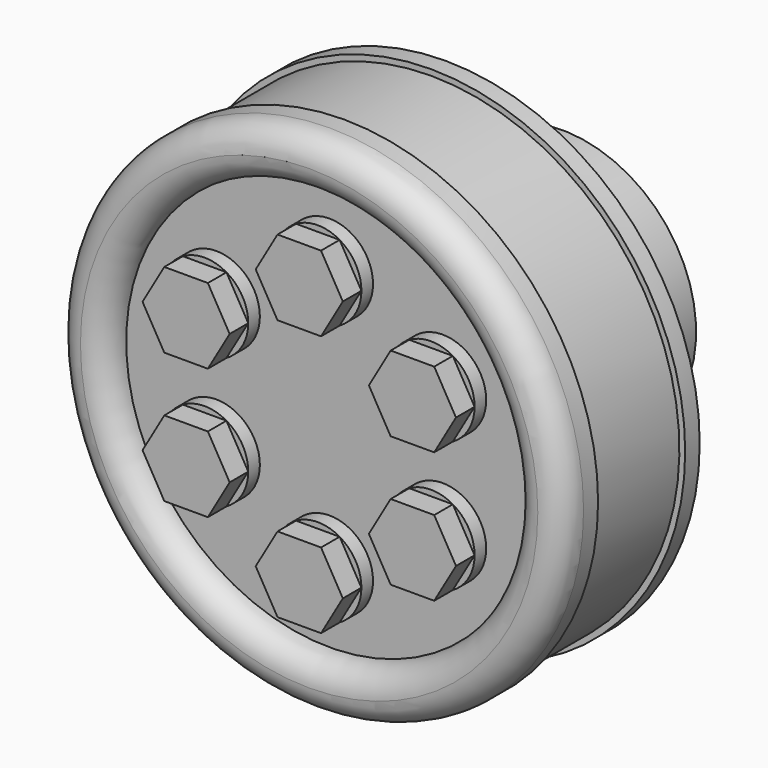
from build123d import *

# Parameters (mm, degrees)
F0_R      = 22.225
F1_DEPTH  = 12.7
F2_R      = 3.81
F3_DEPTH  = 1.27
F5_DEPTH  = 2.032
F6_R      = 22.225
F6_R_2    = 17.78
F7_DEPTH  = 2.2225
F8_R      = 2.22249
F9_R      = 2.2225
F10_R     = 11.7475
F11_DEPTH = 12.7
F12_R     = 3.302
F13_DEPTH = 6.35
F14_R     = 1.7272
F15_DEPTH = 63.5
F16_W     = 9.525
F16_H     = 0.508


# Not quite as in the source:
# - a fillet or chamfer is up to 0.001 mm smaller than in the source, because OpenCascade refuses the exact size


with BuildPart() as f1:
    # F0 (on Front) → F1 (new body)
    with BuildSketch(Plane.XZ):
        Circle(F0_R)
    extrude(amount=F1_DEPTH)

    # F2 (on face) → F3 (join)
    with BuildSketch(Plane.XZ.offset(12.7)):
        with Locations((0, 11.43)):
            Circle(F2_R)
        with Locations((-9.8986703653, 5.715)):
            Circle(F2_R)
        with Locations((-9.8986703653, -5.715)):
            Circle(F2_R)
        with Locations((0, -11.43)):
            Circle(F2_R)
        with Locations((9.8986703653, -5.715)):
            Circle(F2_R)
        with Locations((9.8986703653, 5.715)):
            Circle(F2_R)
    extrude(amount=F3_DEPTH)

    # F4 (on face) → F5 (join)
    with BuildSketch(Plane.XZ.offset(13.97)):
        Polygon((1.905, 8.1304432116), (3.81, 11.43), (1.905, 14.7295567884), (-1.905, 14.7295567884), (-3.81, 11.43), (-1.905, 8.1304432116), align=None)
        Polygon((-7.9936703653, 2.4154432116), (-6.0886703653, 5.715), (-7.9936703653, 9.0145567884), (-11.8036703653, 9.0145567884), (-13.7086703653, 5.715), (-11.8036703653, 2.4154432116), align=None)
        Polygon((7.9936703653, 9.0145567884), (6.0886703653, 5.715), (7.9936703653, 2.4154432116), (11.8036703653, 2.4154432116), (13.7086703653, 5.715), (11.8036703653, 9.0145567884), align=None)
        Polygon((-7.9936703653, -2.4154432116), (-11.8036703653, -2.4154432116), (-13.7086703653, -5.715), (-11.8036703653, -9.0145567884), (-7.9936703653, -9.0145567884), (-6.0886703653, -5.715), align=None)
        Polygon((3.81, -11.43), (1.905, -8.1304432116), (-1.905, -8.1304432116), (-3.81, -11.43), (-1.905, -14.7295567884), (1.905, -14.7295567884), align=None)
        Polygon((7.9936703653, -2.4154432116), (6.0886703653, -5.715), (7.9936703653, -9.0145567884), (11.8036703653, -9.0145567884), (13.7086703653, -5.715), (11.8036703653, -2.4154432116), align=None)
    extrude(amount=F5_DEPTH)

    # F6 (on face) → F7 (join)
    with BuildSketch(Plane.XZ.offset(12.7)):
        Circle(F6_R)
        Circle(F6_R_2, mode=Mode.SUBTRACT)
    extrude(amount=F7_DEPTH)

    # F8 (radius 2.2225 in the source; OpenCascade refuses exactly that, so slightly less here)
    f8_edges = [f1.edges().sort_by_distance(p)[0] for p in [
        (-17.78, -14.9225, 0),
    ]]
    fillet(f8_edges, radius=F8_R)

    # F9
    f9_edges = [f1.edges().sort_by_distance(p)[0] for p in [
        (-22.225, -14.9225, 0),
    ]]
    fillet(f9_edges, radius=F9_R)

    # F10 (on face) → F11 (join)
    with BuildSketch(Plane(origin=(0, 0, 0), x_dir=(-1, 0, 0), z_dir=(0, 1, 0))):
        Circle(F10_R)
    extrude(amount=F11_DEPTH)

    # F12 (on face) → F13 (cut)
    with BuildSketch(Plane(origin=(0, 12.7, 0), x_dir=(-1, 0, 0), z_dir=(0, 1, 0))):
        Circle(F12_R)
    extrude(amount=-F13_DEPTH, mode=Mode.SUBTRACT)

    # F14 (on Top) → F15 (cut, symmetric)
    with BuildSketch(Plane.XY):
        with Locations((0, 5.842)):
            Circle(F14_R)
    extrude(amount=F15_DEPTH, both=True, mode=Mode.SUBTRACT)

    # F16 (on Right) → F18 (revolve, cut)
    with BuildSketch(Plane.YZ):
        with Locations((-6.35, 22.479)):
            Rectangle(F16_W, F16_H)
        with Locations((-6.35, 21.971)):
            Rectangle(F16_W, F16_H)
    revolve(axis=Axis((0, 11.6996625438, 0), (0, 1, 0)), mode=Mode.SUBTRACT)


solid = f1.part
